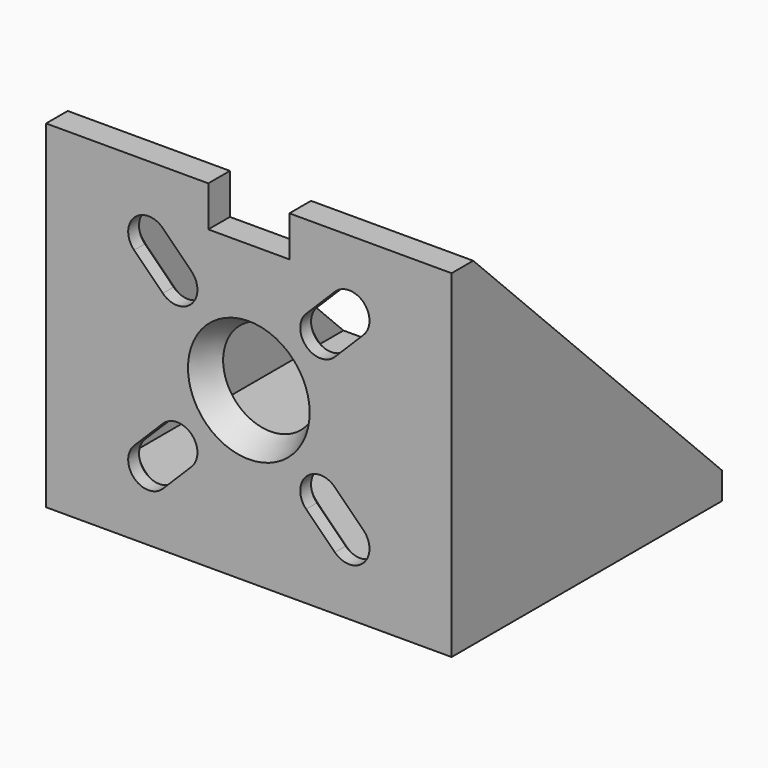
from build123d import *

# Parameters (mm, degrees)
F0_R     = 3.5
F1_DEPTH = 2
F2_W     = 23
F2_H     = 2
F3_DEPTH = 15
F4_START = 13
F4_DEPTH = 2
F5_START = -13
F5_DEPTH = 2
F6_SIZE  = 1
F7_SIZE2 = 0.99999
F7_SIZE  = 1.99999


# Not quite as in the source:
# - a fillet or chamfer is up to 0.001 mm smaller than in the source, because OpenCascade refuses the exact size


with BuildPart() as f1:
    # F0 (on Front) → F1 (new body)
    with BuildSketch(Plane.XZ):
        Polygon((-3, 12.5), (-15, 12.5), (-15, -12.5), (15, -12.5), (15, 12.5), (3, 12.5), (3, 9.5), (-3, 9.5), align=None)
        with BuildLine():
            ThreePointArc((-6.3639610307, -8.4852813742), (-8.4852813742, -8.4852813742), (-8.4852813742, -6.3639610307))
            Line((-8.4852813742, -6.3639610307), (-6.3639610307, -4.2426406871))
            ThreePointArc((-6.3639610307, -4.2426406871), (-4.7292757104, -3.9174815601), (-3.8033008589, -5.3033008589))
            ThreePointArc((-3.8033008589, -5.3033008589), (-3.9174815601, -5.8773260074), (-4.2426406871, -6.3639610307))
            Line((-4.2426406871, -6.3639610307), (-6.3639610307, -8.4852813742))
        make_face(mode=Mode.SUBTRACT)
        with BuildLine():
            ThreePointArc((8.4852813742, -6.3639610307), (8.8104405012, -6.8505960539), (8.9246212025, -7.4246212025))
            ThreePointArc((8.9246212025, -7.4246212025), (7.998646351, -8.8104405012), (6.3639610307, -8.4852813742))
            Line((6.3639610307, -8.4852813742), (4.2426406871, -6.3639610307))
            ThreePointArc((4.2426406871, -6.3639610307), (4.2426406871, -4.2426406871), (6.3639610307, -4.2426406871))
            Line((6.3639610307, -4.2426406871), (8.4852813742, -6.3639610307))
        make_face(mode=Mode.SUBTRACT)
        with BuildLine():
            ThreePointArc((-8.4852813742, 6.3639610307), (-8.4852813742, 8.4852813742), (-6.3639610307, 8.4852813742))
            Line((-6.3639610307, 8.4852813742), (-4.2426406871, 6.3639610307))
            ThreePointArc((-4.2426406871, 6.3639610307), (-3.9174815601, 5.8773260074), (-3.8033008589, 5.3033008589))
            ThreePointArc((-3.8033008589, 5.3033008589), (-4.7292757104, 3.9174815601), (-6.3639610307, 4.2426406871))
            Line((-6.3639610307, 4.2426406871), (-8.4852813742, 6.3639610307))
        make_face(mode=Mode.SUBTRACT)
        Circle(F0_R, mode=Mode.SUBTRACT)
        with BuildLine():
            ThreePointArc((6.3639610307, 8.4852813742), (7.998646351, 8.8104405012), (8.9246212025, 7.4246212025))
            ThreePointArc((8.9246212025, 7.4246212025), (8.8104405012, 6.8505960539), (8.4852813742, 6.3639610307))
            Line((8.4852813742, 6.3639610307), (6.3639610307, 4.2426406871))
            ThreePointArc((6.3639610307, 4.2426406871), (4.2426406871, 4.2426406871), (4.2426406871, 6.3639610307))
            Line((4.2426406871, 6.3639610307), (6.3639610307, 8.4852813742))
        make_face(mode=Mode.SUBTRACT)
    extrude(amount=F1_DEPTH)

    # F2 (on Right) → F3 (join, symmetric)
    with BuildSketch(Plane.YZ):
        with Locations((11.5, -11.5)):
            Rectangle(F2_W, F2_H)
    extrude(amount=F3_DEPTH, both=True)

    # F2 (on Right) → F4 (join)
    with BuildSketch(Plane.YZ.offset(F4_START)):
        Polygon((0, 12.5), (0, -10.5), (23, -10.5), align=None)
    extrude(amount=F4_DEPTH)

    # F2 (on Right) → F5 (join)
    with BuildSketch(Plane.YZ.offset(F5_START)):
        Polygon((0, 12.5), (0, -10.5), (23, -10.5), align=None)
    extrude(amount=-F5_DEPTH)

    # F6
    f6_edges = [f1.edges().sort_by_distance(p)[0] for p in [
        (5.303301, 0, 7.424621),
        (-5.303301, 0, 7.424621),
        (-7.424621, 0, -5.303301),
        (7.424621, 0, -5.303301),
    ]]
    chamfer(f6_edges, length=F6_SIZE)

    # F7 (size 2 and 1 in the source; OpenCascade refuses exactly that, so slightly less here)
    f7_edges = [f1.edges().sort_by_distance(p)[0] for p in [
        (-3.5, -2, 0),
    ]]
    f7_side = f1.faces().sort_by_distance((-3.5, -1, 0))[0]
    chamfer(f7_edges, length=F7_SIZE, length2=F7_SIZE2, reference=f7_side)


solid = f1.part
